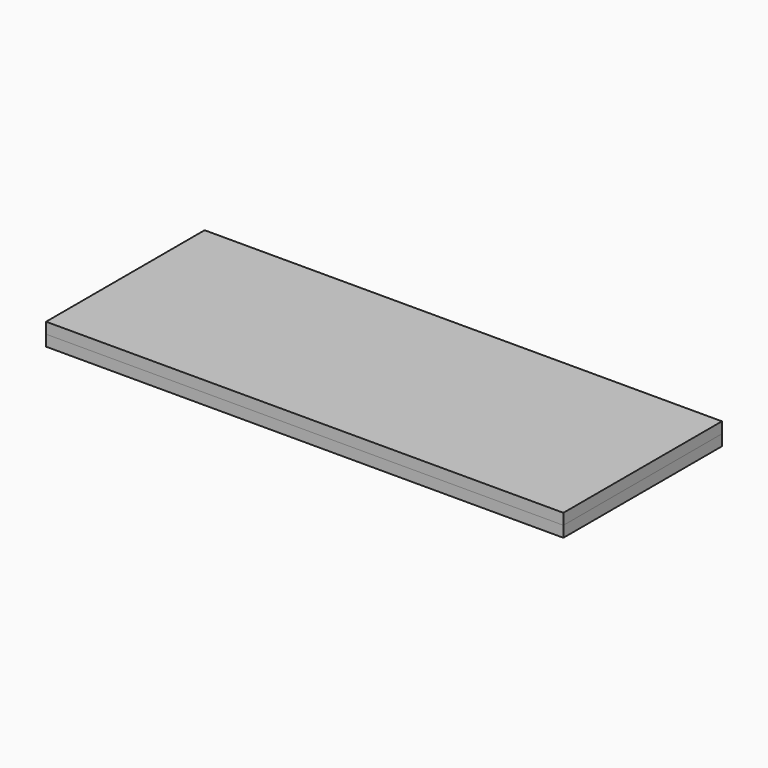
from build123d import *

# Parameters (mm, degrees)
F0_W         = 2
F0_H         = 2
F1_DEPTH     = 1
F2_TEXT_SIZE = 16.1356215055
F3_DEPTH     = 1
F4_W         = 47
F4_H         = 18
F5_DEPTH     = 1


# Not quite as in the source:
# - Text() gives the source's letters only with a copy of the font that has no kerning and outlines rounded to 1/6400 em; it was checked with that copy


with BuildPart() as f1:
    # F0 (on Top) → F1 (new body)
    with BuildSketch(Plane.XY):
        with Locations((22.5, 8)):
            Rectangle(F0_W, F0_H)
        with Locations((-22.5, -8)):
            Rectangle(F0_W, F0_H)
        Polygon((23.5, 7), (21.5, 7), (21.5, -7), (-21.5, -7), (-21.5, -9), (23.5, -9), align=None)
        Polygon((21.5, 9), (-23.5, 9), (-23.5, -7), (-21.5, -7), (-21.5, 7), (21.5, 7), align=None)
    extrude(amount=-F1_DEPTH)


with BuildPart() as f3:
    # F2 (on Top) → F3 (new body)
    with BuildSketch(Plane.XY):
        with Locations((-20.045356825, -5.576162599)):
            Text('AMW', F2_TEXT_SIZE, font='Open Sans', text_align=(TextAlign.LEFT, TextAlign.BOTTOM))
    extrude(amount=-F3_DEPTH)


with BuildPart() as f5:
    # F4 (on Top) → F5 (new body)
    with BuildSketch(Plane.XY):
        Rectangle(F4_W, F4_H)
    extrude(amount=F5_DEPTH)


solid = Compound([f1.part, f3.part, f5.part])
